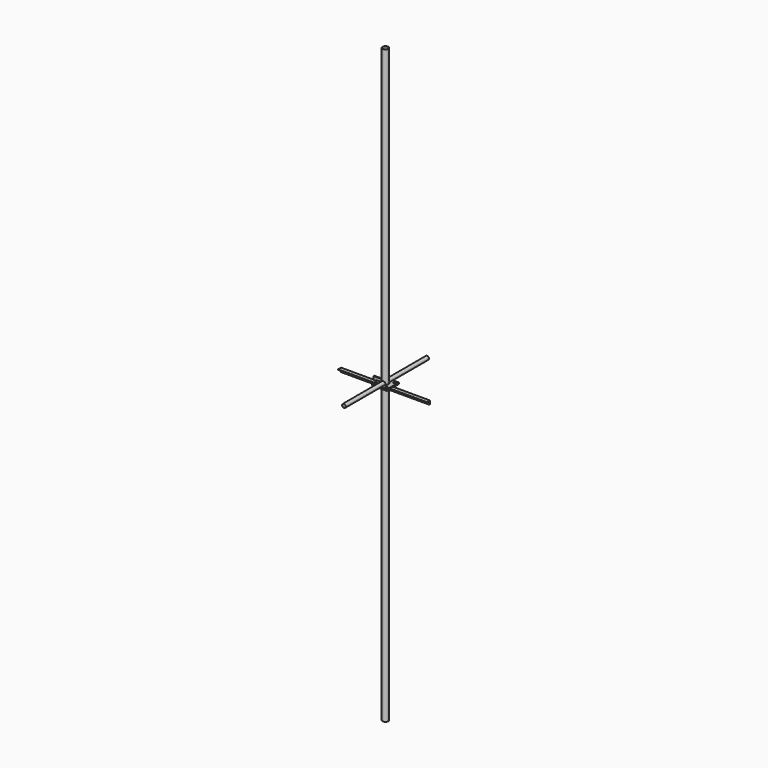
from build123d import *

# Parameters (mm, degrees)
F1_W              = 152.4
F1_H              = 152.4
F1_R              = 11.1125
F1_R_2            = 30.559375
F2_DEPTH          = 7.9375
F3_W              = 90.4875
F3_H              = 69.85
F3_R              = 7.14375
F4_DEPTH          = 4.7625
F5_R              = 30.1625
F5_R_2            = 26.2509
F6_DEPTH          = 3048
F8_DEPTH          = 457.2
F9_R              = 7.14375
F10_DEPTH         = 76.201
F13_DEPTH         = 50.8
F14_R             = 7.14375
F15_DEPTH         = 3048.001
F18_R             = 19.05
F18_R_2           = 17.399
F19_DEPTH         = 400.05
F19_COPIES1_COUNT = 2
F19_COPIES1_PITCH = 135.0645


# Not quite as in the source:
# - a feature of the source that left no trace in its solid (it failed there, or was rolled back) is left out
# - a pattern or mirror of a feature is missing from the dataset's text; its kind, count and spacing are read off the source's solid


with BuildPart() as f2:
    # F1 (on Top) → F2 (new body, symmetric)
    with BuildSketch(Plane.XY):
        Rectangle(F1_W, F1_H)
        with Locations((-50.8, -50.8)):
            Circle(F1_R, mode=Mode.SUBTRACT)
        with Locations((50.8, -50.8)):
            Circle(F1_R, mode=Mode.SUBTRACT)
        with Locations((-50.8, 50.8)):
            Circle(F1_R, mode=Mode.SUBTRACT)
        Circle(F1_R_2, mode=Mode.SUBTRACT)
        with Locations((50.8, 50.8)):
            Circle(F1_R, mode=Mode.SUBTRACT)
    extrude(amount=F2_DEPTH, both=True)


with BuildPart() as f4:
    # F3 (on Front) → F4 (new body, symmetric)
    with BuildSketch(Plane.XZ):
        with Locations((-75.40625, 0)):
            Rectangle(F3_W, F3_H)
        with Locations((-88.9, 0)):
            Circle(F3_R, mode=Mode.SUBTRACT)
    extrude(amount=F4_DEPTH, both=True)


with BuildPart() as f6:
    # F5 (on Top) → F6 (new body, symmetric)
    with BuildSketch(Plane.XY):
        Circle(F5_R)
        Circle(F5_R_2, mode=Mode.SUBTRACT)
    extrude(amount=F6_DEPTH, both=True)


with BuildPart() as f8:
    # F7 (on Right) → F8 (new body, symmetric)
    with BuildSketch(Plane.YZ):
        Polygon((0, 0), (-38.1, 0), (-38.1, -4.7625), (-4.7625, -4.7625), (-4.7625, -38.1), (0, -38.1), align=None)
    extrude(amount=F8_DEPTH, both=True)

    # F9 (on face) → F10 (cut, through all)
    with BuildSketch(Plane(origin=(0, 0, 0), x_dir=(-1, 0, 0), z_dir=(0, 1, 0))):
        with Locations((-431.8, -19.05)):
            Circle(F9_R)
        with Locations((431.8, -19.05)):
            Circle(F9_R)
    extrude(amount=-F10_DEPTH, mode=Mode.SUBTRACT)


with BuildPart() as f13:
    # F12 (on Front) → F13 (new body)
    with BuildSketch(Plane.XZ):
        with BuildLine():
            ThreePointArc((-16.9480915479, 5.9272882453), (-24.5322916182, 6.7362863103), (-20.955, 0))
            Line((-20.955, 0), (20.955, 0))
            ThreePointArc((20.955, 0), (24.5322916182, 6.7362863103), (16.9480915479, 5.9272882453))
            ThreePointArc((16.9480915479, 5.9272882453), (15.5463661286, 4.1908146809), (13.4125840901, 3.5372484617))
            Line((13.4125840901, 3.5372484617), (-13.4125840901, 3.5372484617))
            ThreePointArc((-13.4125840901, 3.5372484617), (-15.5463661286, 4.1908146809), (-16.9480915479, 5.9272882453))
        make_face()
        with BuildLine():
            ThreePointArc((-18.3151544315, 5.3782369616), (-16.3714285168, 2.9703269524), (-13.4125840901, 2.0640484617))
            Line((-13.4125840901, 2.0640484617), (13.4125840901, 2.0640484617))
            ThreePointArc((13.4125840901, 2.0640484617), (16.3714285168, 2.9703269524), (18.3151544315, 5.3782369616))
            ThreePointArc((18.3151544315, 5.3782369616), (23.3118038896, 5.9112239221), (20.955, 1.4732))
            Line((20.955, 1.4732), (-20.955, 1.4732))
            ThreePointArc((-20.955, 1.4732), (-23.3118038896, 5.9112239221), (-18.3151544315, 5.3782369616))
        make_face(mode=Mode.SUBTRACT)
    extrude(amount=F13_DEPTH)

    # F14 (on face) → F15 (cut, through all)
    with BuildSketch(Plane(origin=(0, 0, 0), x_dir=(1, 0, 0), z_dir=(0, 0, -1))):
        with Locations((0, 31.75)):
            Circle(F14_R)
    extrude(amount=-F15_DEPTH, mode=Mode.SUBTRACT)


with BuildPart() as f19:
    # F18 (on Front) → F19 (new body, symmetric)
    with BuildSketch(Plane.XZ):
        with Locations((0, 19.05)):
            Circle(F18_R)
        with Locations((0, 19.05)):
            Circle(F18_R_2, mode=Mode.SUBTRACT)
    extrude(amount=F19_DEPTH, both=True)


with BuildPart() as f19_copies_1:
    # F19_copies: instance of F19
    add(f19.part.mirror(Plane.ZX.offset(67.53225)))

    # F19_copies1: F19 ×2
    with Locations(*[(0, -i * F19_COPIES1_PITCH, 0) for i in range(1, F19_COPIES1_COUNT)]):
        add(f19.part)


solid = Compound([f2.part, f4.part, f6.part, f8.part, f13.part, f19.part, f19_copies_1.part])
